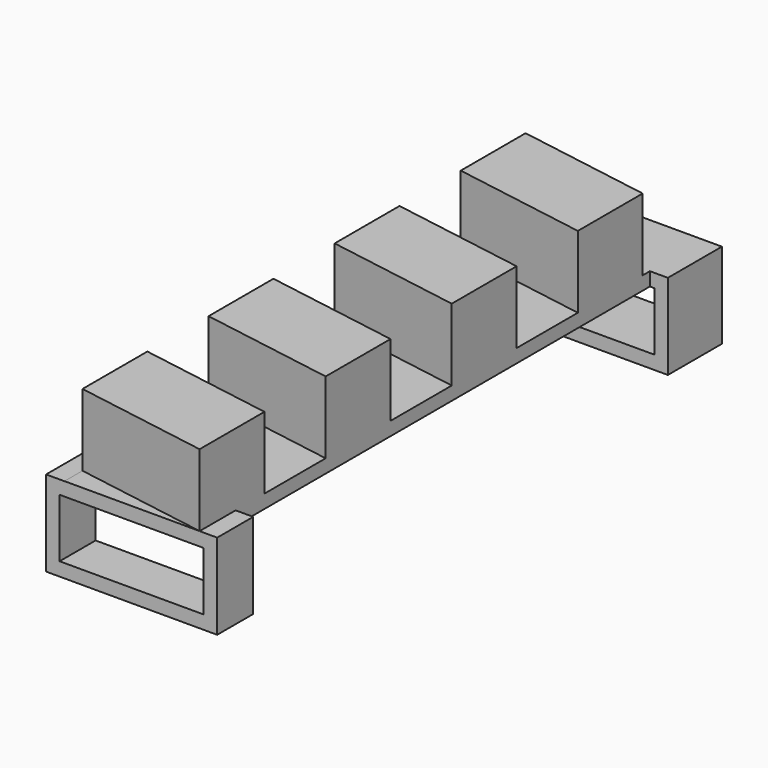
from build123d import *

# Parameters (mm, degrees)
F0_W     = 30
F0_H     = 140
F1_DEPTH = 3
F3_DEPTH = 16
F4_W     = 3
F4_H     = 3
F4_W_2   = 1
F4_W_3   = 30
F4_W_4   = 32
F5_DEPTH = 15
F6_W     = 3
F6_H     = 3
F6_W_2   = 32
F7_DEPTH = 10


with BuildPart() as f1:
    # F0 (on Top) → F1 (new body)
    with BuildSketch(Plane.XY):
        with Locations((27.8885364532, 24.2495501014)):
            Rectangle(F0_W, F0_H)
    extrude(amount=F1_DEPTH)

    # F2 (on face) → F3 (join)
    with BuildSketch(Plane.XY.offset(3)):
        Polygon((42.8885364532, -27.7504498986), (12.8885364532, -22.7504498986), (12.8885364532, -40.7504498986), (42.8885364532, -45.7504498986), align=None)
        Polygon((12.8885364532, 12.2495501014), (12.8885364532, -5.7504498986), (42.8885364532, -10.7504498986), (42.8885364532, 7.2495501014), align=None)
        Polygon((12.8885364532, 47.2495501014), (12.8885364532, 29.2495501014), (42.8885364532, 24.2495501014), (42.8885364532, 42.2495501014), align=None)
        Polygon((12.8885364532, 82.2495501014), (12.8885364532, 64.2495501014), (42.8885364532, 59.2495501014), (42.8885364532, 77.2495501014), align=None)
    extrude(amount=F3_DEPTH)

    # F4 (on face) → F5 (join)
    with BuildSketch(Plane(origin=(0, 94.2495501014, 0), x_dir=(-1, 0, 0), z_dir=(0, 1, 0))):
        with Locations((-45.3885364532, 1.5)):
            Rectangle(F4_W, F4_H)
        with Locations((-43.3885364532, 1.5)):
            Rectangle(F4_W_2, F4_H)
        Polygon((-43.8885364532, 0), (-46.8885364532, 0), (-46.8885364532, -16), (-43.8885364532, -16), (-43.8885364532, -13), align=None)
        with Locations((-27.8885364532, 1.5)):
            Rectangle(F4_W_3, F4_H)
        with Locations((-27.8885364532, -14.5)):
            Rectangle(F4_W_4, F4_H)
        with Locations((-12.3885364532, 1.5)):
            Rectangle(F4_W_2, F4_H)
        Polygon((-11.8885364532, 0), (-11.8885364532, -13), (-11.8885364532, -16), (-8.8885364532, -16), (-8.8885364532, 0), align=None)
        with Locations((-10.3885364532, 1.5)):
            Rectangle(F4_W, F4_H)
    extrude(amount=-F5_DEPTH)

    # F6 (on face) → F7 (join)
    with BuildSketch(Plane.XZ.offset(45.7504498986)):
        with Locations((10.2999972403, 1.4885346591)):
            Rectangle(F6_W, F6_H)
        Polygon((11.7999972403, -0.0114653409), (8.7999972403, -0.0114653409), (8.7999972403, -16.0114653409), (11.7999972403, -16.0114653409), (11.7999972403, -13.0114653409), align=None)
        with Locations((27.7999972403, -14.5114653409)):
            Rectangle(F6_W_2, F6_H)
        Polygon((46.7999972403, -0.0114653409), (43.7999972403, -0.0114653409), (43.7999972403, -13.0114653409), (43.7999972403, -16.0114653409), (46.7999972403, -16.0114653409), align=None)
        with Locations((45.2999972403, 1.4885346591)):
            Rectangle(F6_W, F6_H)
        Polygon((12.8885364532, 2.9885346591), (11.7999972403, 2.9885346591), (11.7999972403, -0.0114653409), (43.7999972403, -0.0114653409), (43.7999972403, 2.9885346591), (42.8885364532, 2.9885346591), (42.8885364532, 0), (12.8885364532, 0), align=None)
    extrude(amount=-F7_DEPTH)


solid = f1.part
